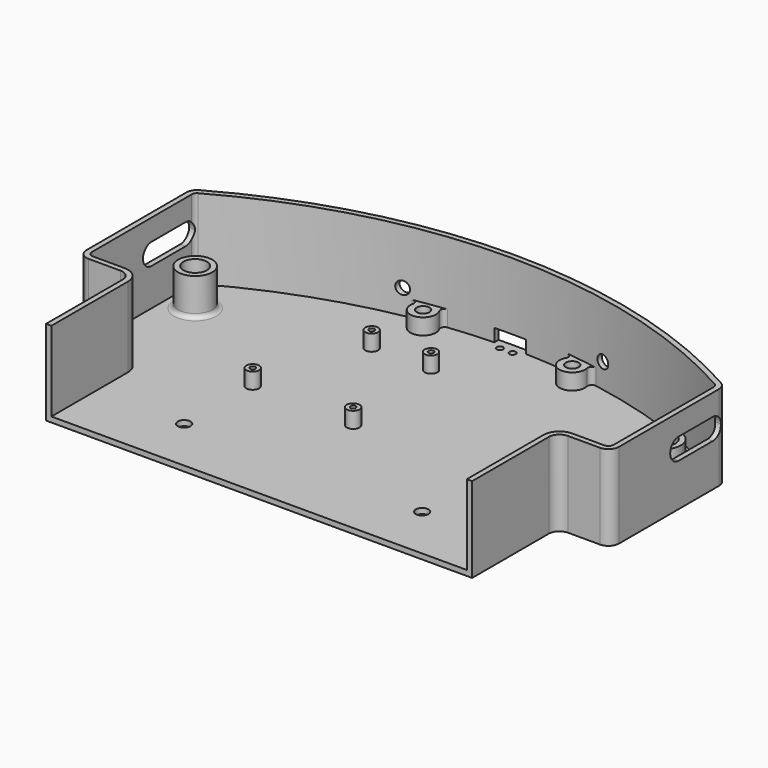
from build123d import *

# Parameters (mm, degrees)
F1_DEPTH       = 40
F2_W           = 100
F2_H           = 200
F3_DEPTH       = 100
F4_R           = 5
F5_T           = -2.5
F6_R           = 3
F7_DEPTH       = 25
F8_R           = 8
F9_DEPTH       = 25
F10_R          = 5.5
F11_DEPTH      = 25
F12_R          = 3
F12_R_2        = 1.25
F13_DEPTH      = 10
F14_R          = 3
F15_DEPTH      = 150
F17_START      = -41.94633
F16_W          = 15
F16_H          = 6
F17_DEPTH      = 208.05367
F18_R          = 1.5
F19_DEPTH      = 12.5
F20_R          = 6
F21_DEPTH      = 0.01
F21_DEPTH_BACK = 10
F22_R          = 3
F23_DEPTH      = 12.5
F24_R          = 2
F26_DEPTH      = 150


with BuildPart() as f1:
    # F0 (on Top) → F1 (new body)
    with BuildSketch(Plane.XY):
        with BuildLine():
            Line((-125, 66.5063509461), (-125, -50))
            Line((-125, -50), (125, -50))
            Line((125, -50), (125, 66.5063509461))
            ThreePointArc((125, 66.5063509461), (64.7047614336, 91.4814565299), (3.27e-07, 100))
            ThreePointArc((3.27e-07, 100), (-64.7047611177, 91.4814566146), (-125, 66.5063509461))
        make_face()
    extrude(amount=F1_DEPTH)

    # F2 (on Top) → F3 (cut)
    with BuildSketch(Plane.XY):
        with Locations((-150, -100)):
            Rectangle(F2_W, F2_H)
        with Locations((150, -100)):
            Rectangle(F2_W, F2_H)
    extrude(amount=F3_DEPTH, mode=Mode.SUBTRACT)

    # F4
    f4_edges = [f1.edges().sort_by_distance(p)[0] for p in [
        (-125, 66.506351, 20),
        (125, 66.506351, 20),
        (125, 0, 20),
        (100, 0, 20),
        (-125, 0, 20),
        (-100, 0, 20),
    ]]
    fillet(f4_edges, radius=F4_R)

    # F5
    f5_openings = [f1.faces().sort_by_distance(p)[0] for p in [
        (0, 23.401227, 40),
        (0, -50, 20),
    ]]
    offset(amount=F5_T, openings=f5_openings)

    # F6 (on Top) → F7 (cut)
    with BuildSketch(Plane.XY):
        with Locations((-55.8614357137, -24.1385642863)):
            Circle(F6_R)
        with Locations((55.8614357137, -24.1385642863)):
            Circle(F6_R)
    extrude(amount=F7_DEPTH, mode=Mode.SUBTRACT)

    # F8 (on Top) → F9 (join)
    with BuildSketch(Plane.XY):
        with Locations((-110, 50)):
            Circle(F8_R)
        with Locations((110, 50)):
            Circle(F8_R)
    extrude(amount=F9_DEPTH)

    # F10 (on Top) → F11 (cut)
    with BuildSketch(Plane.XY):
        with Locations((-110, 50)):
            Circle(F10_R)
        with Locations((110, 50)):
            Circle(F10_R)
    extrude(amount=F11_DEPTH, mode=Mode.SUBTRACT)

    # F12 (on Top) → F13 (join)
    with BuildSketch(Plane.XY):
        with Locations((-55, 15)):
            Circle(F12_R)
        with Locations((-55, 15)):
            Circle(F12_R_2, mode=Mode.SUBTRACT)
        with Locations((-39.8, 65.8)):
            Circle(F12_R)
        with Locations((-39.8, 65.8)):
            Circle(F12_R_2, mode=Mode.SUBTRACT)
        with Locations((-11.9, 65.8)):
            Circle(F12_R)
        with Locations((-11.9, 65.8)):
            Circle(F12_R_2, mode=Mode.SUBTRACT)
        with Locations((-6.8, 13.7)):
            Circle(F12_R)
        with Locations((-6.8, 13.7)):
            Circle(F12_R_2, mode=Mode.SUBTRACT)
    extrude(amount=F13_DEPTH)

    # F14 (on Front) → F15 (cut, symmetric)
    with BuildSketch(Plane.XZ):
        with Locations((47, 14)):
            Circle(F14_R)
        with Locations((-47, 14)):
            Circle(F14_R)
    extrude(amount=F15_DEPTH, both=True, mode=Mode.SUBTRACT)

    # F16 (on Front) → F17 (cut)
    with BuildSketch(Plane.XZ.offset(F17_START)):
        with Locations((0, 5.5)):
            Rectangle(F16_W, F16_H)
    extrude(amount=-F17_DEPTH, mode=Mode.SUBTRACT)

    # F18 (on Top) → F19 (cut, symmetric)
    with BuildSketch(Plane.XY):
        with Locations((-3, 95)):
            Circle(F18_R)
        with Locations((3, 95)):
            Circle(F18_R)
    extrude(amount=F19_DEPTH, both=True, mode=Mode.SUBTRACT)

    # F20 (on Top) → F21 (join, two sides)
    with BuildSketch(Plane.XY) as f21_sk:
        with Locations((-35, 90)):
            Circle(F20_R)
        with Locations((35, 90)):
            Circle(F20_R)
    extrude(amount=-F21_DEPTH)
    extrude(f21_sk.sketch, amount=F21_DEPTH_BACK)

    # F22 (on face) → F23 (cut, symmetric)
    with BuildSketch(Plane(origin=(0, 0, 0), x_dir=(1, 0, 0), z_dir=(0, 0, -1))):
        with Locations((-35, -90)):
            Circle(F22_R)
        with Locations((35, -90)):
            Circle(F22_R)
    extrude(amount=F23_DEPTH, both=True, mode=Mode.SUBTRACT)

    # F24
    f24_edges = [f1.edges().sort_by_distance(p)[0] for p in [
        (-32.339812, 95.378048, 6.25),
        (-39.085326, 94.394328, 6.25),
        (39.085326, 94.394328, 6.25),
        (32.339812, 95.378048, 6.25),
        (-118, 50, 2.5),
        (102, 50, 2.5),
    ]]
    fillet(f24_edges, radius=F24_R)

    # F25 (on Right) → F26 (cut, symmetric)
    with BuildSketch(Plane.YZ):
        with BuildLine():
            Line((40, 20), (40, 30))
            ThreePointArc((40, 30), (35, 25), (40, 20))
        make_face()
        with BuildLine():
            ThreePointArc((65, 25), (63.5355339059, 28.5355339059), (60, 30))
            Line((60, 30), (60, 20))
            ThreePointArc((60, 20), (63.5355339059, 21.4644660941), (65, 25))
        make_face()
        with BuildLine():
            Line((60, 30), (40, 30))
            ThreePointArc((40, 30), (43.5355339059, 28.5355339059), (45, 25))
            ThreePointArc((45, 25), (43.5355339059, 21.4644660941), (40, 20))
            Line((40, 20), (60, 20))
            ThreePointArc((60, 20), (55, 25), (60, 30))
        make_face()
        with BuildLine():
            ThreePointArc((45, 25), (43.5355339059, 28.5355339059), (40, 30))
            Line((40, 30), (40, 20))
            ThreePointArc((40, 20), (43.5355339059, 21.4644660941), (45, 25))
        make_face()
        with BuildLine():
            Line((60, 20), (60, 30))
            ThreePointArc((60, 30), (55, 25), (60, 20))
        make_face()
    extrude(amount=F26_DEPTH, both=True, mode=Mode.SUBTRACT)


solid = f1.part
